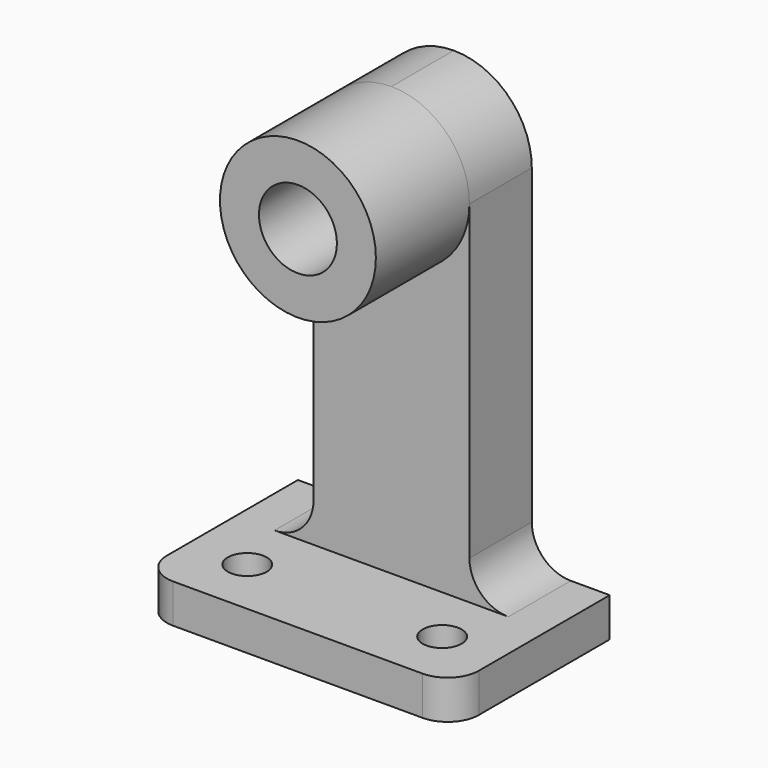
from build123d import *

# Parameters (mm, degrees)
F0_W      = 50.8
F0_H      = 31.75
F1_DEPTH  = 6.35
F2_R      = 3.175
F3_DEPTH  = 6.35
F4_W      = 25.4
F4_H      = 69.85
F5_DEPTH  = 12.7
F7_DEPTH  = 25.4
F8_R      = 12.7
F9_DEPTH  = 19.05
F10_R     = 6.35
F11_DEPTH = 31.75
F12_R     = 5.08
F13_W     = 12.7
F13_H     = 12.7
F14_DEPTH = 12.7
F16_DEPTH = 25.4
F17_W     = 12.7
F17_H     = 12.7
F18_DEPTH = 12.7
F20_DEPTH = 25.4


with BuildPart() as f1:
    # F0 (on Top) → F1 (new body)
    with BuildSketch(Plane.XY):
        with Locations((25.4, 15.875)):
            Rectangle(F0_W, F0_H)
    extrude(amount=F1_DEPTH)

    # F2 (on face) → F3 (cut)
    with BuildSketch(Plane.XY.offset(6.35)):
        with Locations((41.275, 9.525)):
            Circle(F2_R)
        with Locations((9.525, 9.525)):
            Circle(F2_R)
    extrude(amount=-F3_DEPTH, mode=Mode.SUBTRACT)

    # F4 (on face) → F5 (join)
    with BuildSketch(Plane(origin=(0, 31.75, 0), x_dir=(-1, 0, 0), z_dir=(0, 1, 0))):
        with Locations((-25.4, 41.275)):
            Rectangle(F4_W, F4_H)
    extrude(amount=-F5_DEPTH)

    # F6 (on face) → F7 (cut)
    with BuildSketch(Plane.XZ.offset(-19.05)):
        with BuildLine():
            ThreePointArc((25.4, 76.2), (34.3802561211, 72.4802561211), (38.1, 63.5))
            Line((38.1, 63.5), (38.1, 76.2))
            Line((38.1, 76.2), (25.4, 76.2))
        make_face()
        with BuildLine():
            ThreePointArc((12.7, 63.5), (16.4197438789, 72.4802561211), (25.4, 76.2))
            Line((25.4, 76.2), (12.7, 76.2))
            Line((12.7, 76.2), (12.7, 63.5))
        make_face()
    extrude(amount=-F7_DEPTH, mode=Mode.SUBTRACT)

    # F8 (on face) → F9 (join)
    with BuildSketch(Plane.XZ.offset(-19.05)):
        with Locations((25.4, 63.5)):
            Circle(F8_R)
    extrude(amount=F9_DEPTH)

    # F10 (on face) → F11 (cut)
    with BuildSketch(Plane.XZ):
        with Locations((25.4, 63.5)):
            Circle(F10_R)
    extrude(amount=-F11_DEPTH, mode=Mode.SUBTRACT)

    # F12
    f12_edges = [f1.edges().sort_by_distance(p)[0] for p in [
        (0, 0, 3.175),
        (50.8, 0, 3.175),
    ]]
    fillet(f12_edges, radius=F12_R)

    # F13 (on face) → F14 (join)
    with BuildSketch(Plane.YZ.offset(38.1)):
        with Locations((25.4, 12.7)):
            Rectangle(F13_W, F13_H)
    extrude(amount=F14_DEPTH)

    # F15 (on face) → F16 (cut)
    with BuildSketch(Plane.XZ.offset(-19.05)):
        with BuildLine():
            ThreePointArc((38.1, 12.7), (44.45, 6.35), (50.8, 12.7))
            ThreePointArc((50.8, 12.7), (44.45, 19.05), (38.1, 12.7))
        make_face()
        with BuildLine():
            Line((50.8, 19.05), (44.45, 19.05))
            ThreePointArc((44.45, 19.05), (48.9401280605, 17.1901280605), (50.8, 12.7))
            Line((50.8, 12.7), (50.8, 19.05))
        make_face()
        with BuildLine():
            Line((44.45, 19.05), (38.1, 19.05))
            Line((38.1, 19.05), (38.1, 12.7))
            ThreePointArc((38.1, 12.7), (39.9598719395, 17.1901280605), (44.45, 19.05))
        make_face()
        with BuildLine():
            ThreePointArc((50.8, 12.7), (48.9401280605, 8.2098719395), (44.45, 6.35))
            Line((44.45, 6.35), (50.8, 6.35))
            Line((50.8, 6.35), (50.8, 12.7))
        make_face()
    extrude(amount=-F16_DEPTH, mode=Mode.SUBTRACT)

    # F17 (on face) → F18 (join)
    with BuildSketch(Plane(origin=(12.7, 0, 0), x_dir=(0, -1, 0), z_dir=(-1, 0, 0))):
        with Locations((-25.4, 12.7)):
            Rectangle(F17_W, F17_H)
    extrude(amount=F18_DEPTH)

    # F19 (on face) → F20 (cut)
    with BuildSketch(Plane.XZ.offset(-19.05)):
        with BuildLine():
            ThreePointArc((6.35, 6.35), (10.8401280605, 8.2098719395), (12.7, 12.7))
            ThreePointArc((12.7, 12.7), (10.8401280605, 17.1901280605), (6.35, 19.05))
            ThreePointArc((6.35, 19.05), (1.8598719395, 17.1901280605), (0, 12.7))
            ThreePointArc((0, 12.7), (1.8598719395, 8.2098719395), (6.35, 6.35))
        make_face()
        with BuildLine():
            ThreePointArc((0, 12.7), (1.8598719395, 17.1901280605), (6.35, 19.05))
            Line((6.35, 19.05), (0, 19.05))
            Line((0, 19.05), (0, 12.7))
        make_face()
        with BuildLine():
            Line((0, 6.35), (6.35, 6.35))
            ThreePointArc((6.35, 6.35), (1.8598719395, 8.2098719395), (0, 12.7))
            Line((0, 12.7), (0, 6.35))
        make_face()
        with BuildLine():
            Line((12.7, 12.7), (12.7, 19.05))
            Line((12.7, 19.05), (6.35, 19.05))
            ThreePointArc((6.35, 19.05), (10.8401280605, 17.1901280605), (12.7, 12.7))
        make_face()
    extrude(amount=-F20_DEPTH, mode=Mode.SUBTRACT)


solid = f1.part
